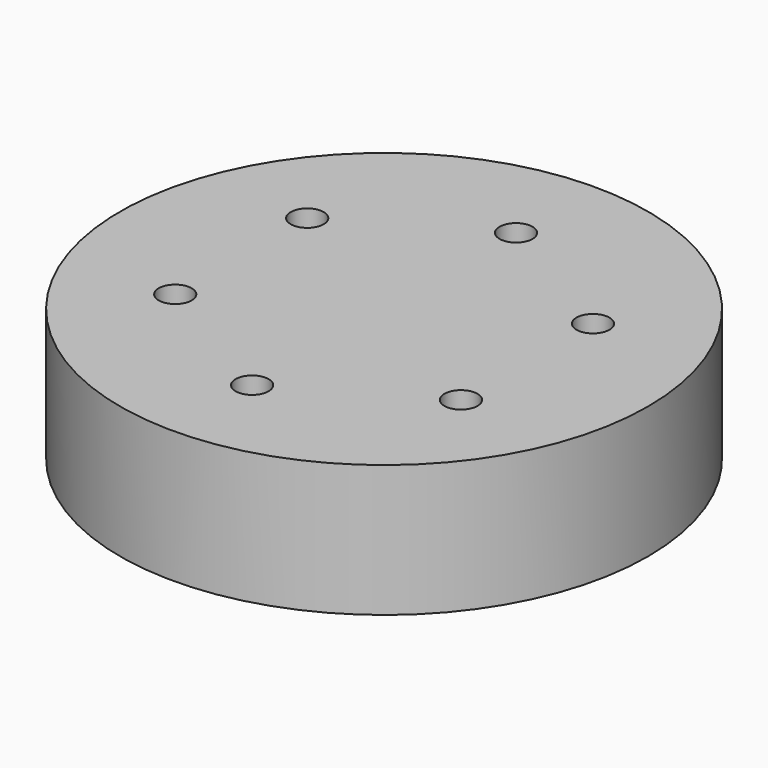
from build123d import *

# Parameters (mm, degrees)
F0_R            = 50.8
F1_DEPTH        = 25.4
F2_R            = 3.175
F3_DEPTH        = 25.401
F3_COPIES_COUNT = 6


# Not quite as in the source:
# - a pattern or mirror of a feature is missing from the dataset's text; its kind, count and spacing are read off the source's solid


with BuildPart() as f1:
    # F0 (on Top) → F1 (new body)
    with BuildSketch(Plane.XY):
        Circle(F0_R)
    extrude(amount=F1_DEPTH)

    # F2 (on face) → F3 (cut, through all)
    with BuildSketch(Plane.XY.offset(25.4)):
        with Locations((0, -31.75)):
            Circle(F2_R)
    f3 = extrude(amount=-F3_DEPTH, mode=Mode.SUBTRACT)

    # F3_copies: F3 ×6 about axis
    f3_copies_axis = Axis((0, 0, 0), (0, 0, 1))
    for i in range(1, F3_COPIES_COUNT):
        add(f3.rotate(f3_copies_axis, i * 360 / F3_COPIES_COUNT), mode=Mode.SUBTRACT)


solid = f1.part
